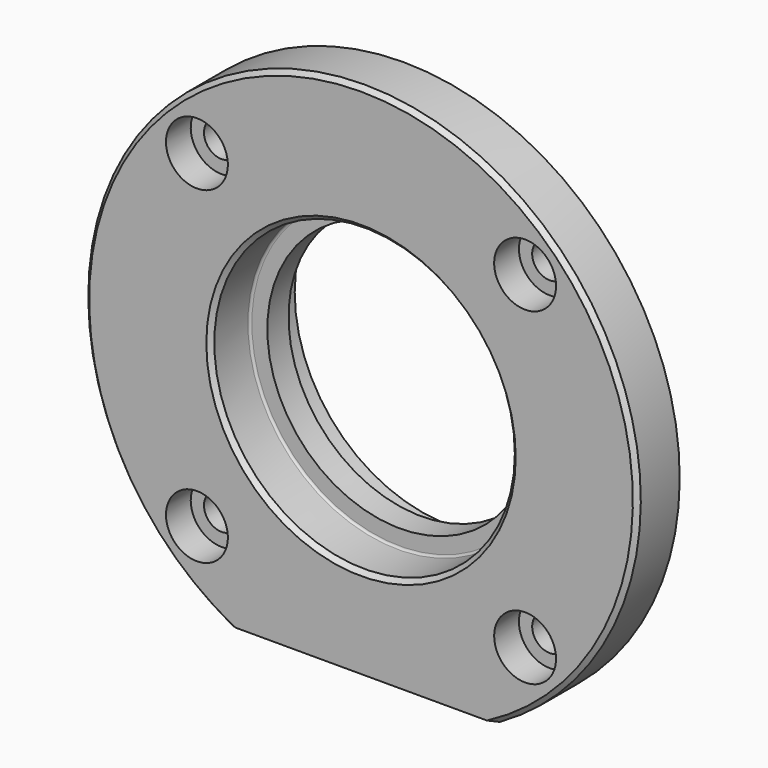
from build123d import *

# Parameters (mm, degrees)
F0_R            = 62.5
F1_DEPTH        = 12
F2_R            = 7
F3_DEPTH        = 7
F3_COPIES_COUNT = 4
F4_R            = 4
F5_DEPTH        = 25
F5_COPIES_COUNT = 4
F7_DEPTH        = 25
F8_R            = 42.5
F9_DEPTH        = 13
F10_R           = 35
F11_DEPTH       = 8
F12_R           = 34
F13_DEPTH       = 11
F14_R           = 30
F15_DEPTH       = 25
F16_SIZE        = 1
F17_R           = 0.5
F18_R           = 3


# Not quite as in the source:
# - a pattern or mirror of a feature is missing from the dataset's text; its kind, count and spacing are read off the source's solid


with BuildPart() as f1:
    # F0 (on Front) → F1 (new body)
    with BuildSketch(Plane.XZ):
        Circle(F0_R)
    extrude(amount=-F1_DEPTH)

    # F2 (on face) → F3 (cut)
    with BuildSketch(Plane.XZ):
        with Locations((37.1231060123, 37.1231060123)):
            Circle(F2_R)
    f3 = extrude(amount=-F3_DEPTH, mode=Mode.SUBTRACT)

    # F3_copies: F3 ×4 about axis
    f3_copies_axis = Axis((0, 0, 0), (0, 1, 0))
    for i in range(1, F3_COPIES_COUNT):
        add(f3.rotate(f3_copies_axis, i * 360 / F3_COPIES_COUNT), mode=Mode.SUBTRACT)

    # F4 (on face) → F5 (cut)
    with BuildSketch(Plane.XZ.offset(-7)):
        with Locations((37.1231060123, 37.1231060123)):
            Circle(F4_R)
    f5 = extrude(amount=-F5_DEPTH, mode=Mode.SUBTRACT)

    # F5_copies: F5 ×4 about axis
    f5_copies_axis = Axis((0, 0, 0), (0, 1, 0))
    for i in range(1, F5_COPIES_COUNT):
        add(f5.rotate(f5_copies_axis, i * 360 / F5_COPIES_COUNT), mode=Mode.SUBTRACT)

    # F6 (on face) → F7 (cut)
    with BuildSketch(Plane.XZ):
        with BuildLine():
            Line((30.5941170816, -54.5), (-30.5941170816, -54.5))
            ThreePointArc((-30.5941170816, -54.5), (0, -62.5), (30.5941170816, -54.5))
        make_face()
    extrude(amount=-F7_DEPTH, mode=Mode.SUBTRACT)

    # F8 (on face) → F9 (join)
    with BuildSketch(Plane(origin=(0, 12, 0), x_dir=(-1, 0, 0), z_dir=(0, 1, 0))):
        Circle(F8_R)
    extrude(amount=F9_DEPTH)

    # F10 (on face) → F11 (cut)
    with BuildSketch(Plane(origin=(0, 25, 0), x_dir=(-1, 0, 0), z_dir=(0, 1, 0))):
        Circle(F10_R)
    extrude(amount=-F11_DEPTH, mode=Mode.SUBTRACT)

    # F12 (on face) → F13 (cut)
    with BuildSketch(Plane.XZ):
        Circle(F12_R)
    extrude(amount=-F13_DEPTH, mode=Mode.SUBTRACT)

    # F14 (on face) → F15 (cut)
    with BuildSketch(Plane.XZ.offset(-11)):
        Circle(F14_R)
    extrude(amount=-F15_DEPTH, mode=Mode.SUBTRACT)

    # F16
    f16_edges = [f1.edges().sort_by_distance(p)[0] for p in [
        (0, 0, 62.5),
        (-34, 0, 0),
        (42.5, 25, 0),
    ]]
    chamfer(f16_edges, length=F16_SIZE)

    # F17
    f17_edges = [f1.edges().sort_by_distance(p)[0] for p in [
        (-34, 11, 0),
        (42.5, 12, 0),
    ]]
    fillet(f17_edges, radius=F17_R)

    # F18
    f18_edges = [f1.edges().sort_by_distance(p)[0] for p in [
        (35, 17, 0),
    ]]
    fillet(f18_edges, radius=F18_R)


with BuildPart() as f20:
    # F19 (on Top) → F20 (revolve)
    with BuildSketch(Plane.XY):
        with BuildLine():
            Line((23, 17), (23, 0))
            Line((23, 0), (34, 0))
            Line((34, 0), (34, 10.5))
            ThreePointArc((34, 10.5), (33.8535533906, 10.8535533906), (33.5, 11))
            Line((33.5, 11), (30, 11))
            Line((30, 11), (30, 17))
            Line((30, 17), (23, 17))
        make_face()
    revolve(axis=Axis((0, 0, 0), (0, -1, 0)))


solid = f1.part
